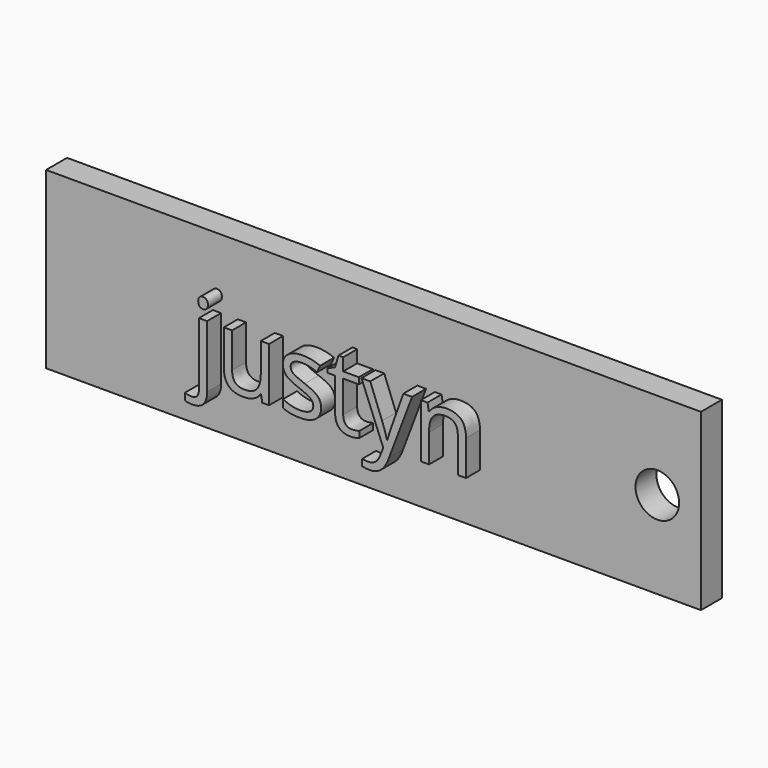
from build123d import *

# Parameters (mm, degrees)
F0_W         = 75
F0_H         = 20
F0_R         = 2.5
F1_DEPTH     = 3
F2_TEXT_SIZE = 11.5505063958
F3_DEPTH     = 2


# Not quite as in the source:
# - Text() gives the source's letters only with a copy of the font that has no kerning and outlines rounded to 1/6400 em; it was checked with that copy


with BuildPart() as f1:
    # F0 (on Front) → F1 (new body)
    with BuildSketch(Plane.XZ):
        with Locations((37.5, -10)):
            Rectangle(F0_W, F0_H)
        with Locations((70, -10)):
            Circle(F0_R, mode=Mode.SUBTRACT)
    extrude(amount=F1_DEPTH)

    # F2 (on face) → F3 (join)
    with BuildSketch(Plane.XZ.offset(3)):
        with Locations((18.1112196296, -14.097915031)):
            Text('justyn', F2_TEXT_SIZE, font='Open Sans', text_align=(TextAlign.LEFT, TextAlign.BOTTOM))
    extrude(amount=F3_DEPTH)


solid = f1.part
